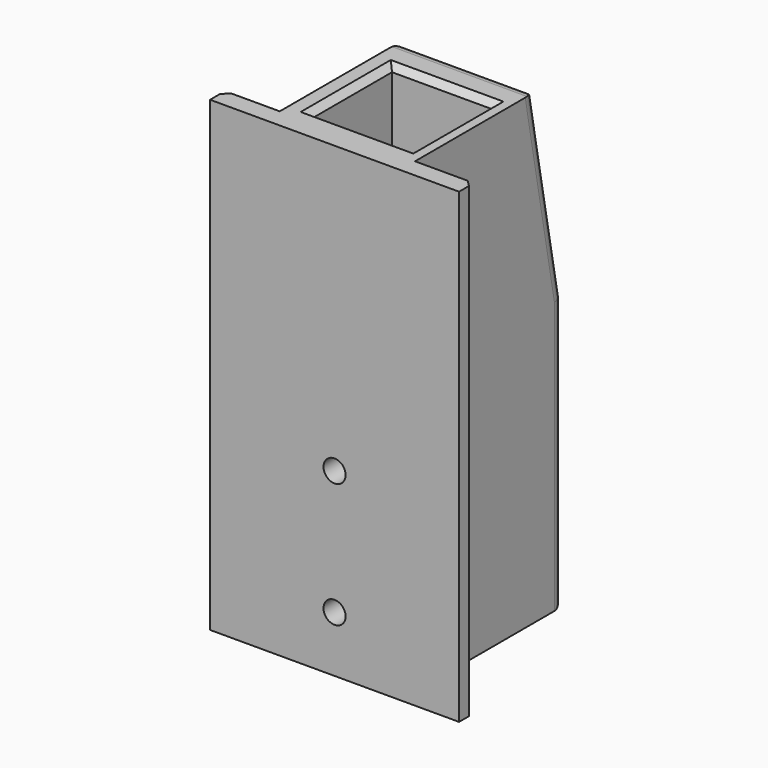
from build123d import *

# Parameters (mm, degrees)
F0_W          = 21.733042784
F0_H          = 30
F0_W_2        = 16.1
F0_H_2        = 16.1
F1_DEPTH      = 75
F2_W          = 20
F2_H          = 3
F3_DEPTH      = 10
F3_DEPTH_BACK = 10
F4_R          = 1.775
F5_DEPTH      = 0.25
F6_R          = 1.775
F7_DEPTH      = 40
F8_SIZE       = 1
F9_SIZE       = 1
F11_DEPTH     = 45.4
F12_R         = 2
F13_TEXT_SIZE = 6.9860524187
F14_DEPTH     = 0.25


# Not quite as in the source:
# - Text() gives the source's letters only with a copy of the font that has no kerning and outlines rounded to 1/6400 em; it was checked with that copy


with BuildPart() as f1:
    # F0 (on Top) → F1 (new body)
    with BuildSketch(Plane.XY):
        with Locations((-0.3418945707, 4.45)):
            Rectangle(F0_W, F0_H)
        Rectangle(F0_W_2, F0_H_2, mode=Mode.SUBTRACT)
        Polygon((10.5246268213, -10.55), (-11.2084159628, -10.55), (-20, -10.55), (-20, -13.55), (20, -13.55), (20, -10.55), align=None)
    extrude(amount=F1_DEPTH)

    # F2 (on Right) → F3 (join, two sides)
    with BuildSketch(Plane.YZ) as f3_sk:
        with Locations((0, 1.5)):
            Rectangle(F2_W, F2_H)
    extrude(amount=F3_DEPTH)
    extrude(f3_sk.sketch, amount=-F3_DEPTH_BACK)

    # F4 (on face) → F5 (cut)
    with BuildSketch(Plane(origin=(0, -10.55, 0), x_dir=(-1, 0, 0), z_dir=(0, 1, 0))):
        with Locations((-15.5, 4.5)):
            Circle(F4_R)
        with Locations((15.5, 4.5)):
            Circle(F4_R)
        with Locations((-15.5, 70.5)):
            Circle(F4_R)
        with Locations((15.5, 70.5)):
            Circle(F4_R)
    extrude(amount=-F5_DEPTH, mode=Mode.SUBTRACT)

    # F6 (on face) → F7 (cut)
    with BuildSketch(Plane(origin=(0, 19.45, 0), x_dir=(-1, 0, 0), z_dir=(0, 1, 0))):
        with Locations((0, 9)):
            Circle(F6_R)
        with Locations((0, 29)):
            Circle(F6_R)
    extrude(amount=-F7_DEPTH, mode=Mode.SUBTRACT)

    # F8
    f8_edges = [f1.edges().sort_by_distance(p)[0] for p in [
        (-8.05, 0, 75),
        (0, 8.05, 75),
        (8.05, 0, 75),
        (0, -8.05, 75),
    ]]
    chamfer(f8_edges, length=F8_SIZE)

    # F9
    f9_edges = [f1.edges().sort_by_distance(p)[0] for p in [
        (20, -10.55, 37.5),
        (-20, -10.55, 37.5),
    ]]
    chamfer(f9_edges, length=F9_SIZE)

    # F10 (on face) → F11 (cut)
    with BuildSketch(Plane.YZ.offset(10.5246268213)):
        Polygon((13.6245964095, 75), (19.45, 43.8646972179), (19.45, 75), align=None)
    extrude(amount=-F11_DEPTH, mode=Mode.SUBTRACT)

    # F12
    f12_edges = [f1.edges().sort_by_distance(p)[0] for p in [
        (10.524627, 19.45, 21.932349),
        (10.524627, 16.537298, 59.432349),
        (-0.341895, 19.45, 43.864697),
        (-11.208416, 19.45, 21.932349),
        (-0.341895, 19.45, 0),
        (-11.208416, 16.537298, 59.432349),
        (-0.341895, 13.624596, 75),
    ]]
    fillet(f12_edges, radius=F12_R)

    # F13 (on face) → F14 (cut)
    with BuildSketch(Plane(origin=(0, 26.7216434687, 4.9996095717), x_dir=(-1, 0, 0), z_dir=(0, 0.9829433965, 0.1839083445))):
        with Locations(Location((-7.1508060209, 68.0241845548), (0, 0, -90))):
            Text('kk', F13_TEXT_SIZE, font='Open Sans', font_style=FontStyle.BOLD, text_align=(TextAlign.LEFT, TextAlign.BOTTOM))
    extrude(amount=-F14_DEPTH, mode=Mode.SUBTRACT)


solid = f1.part
